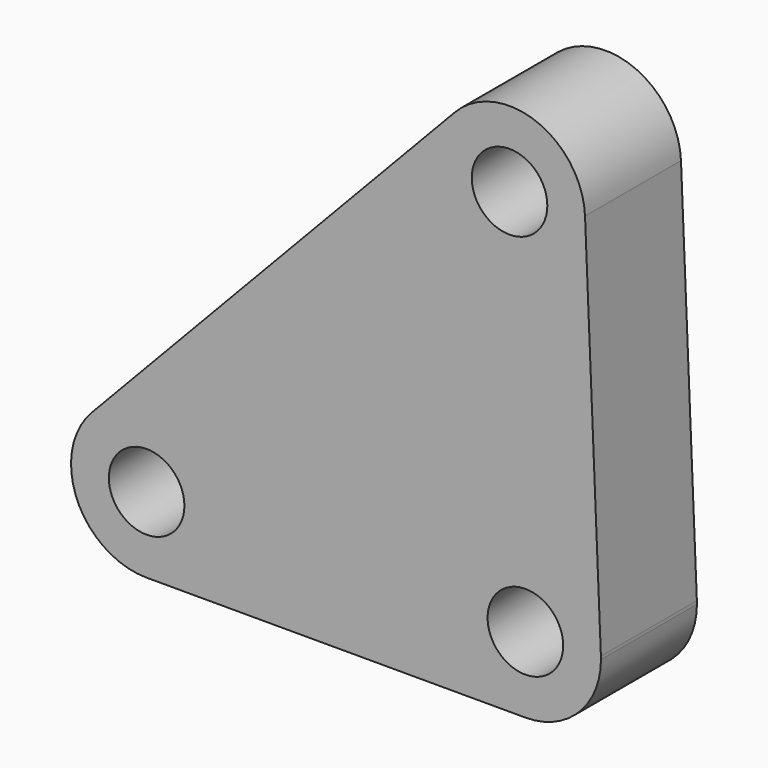
from build123d import *

# Parameters (mm, degrees)
F1_DEPTH = 12.7
F2_R     = 4.0005
F2_R_2   = 4
F3_DEPTH = 12.7


with BuildPart() as f1:
    # F0 (on Front) → F1 (new body)
    with BuildSketch(Plane.XZ):
        with BuildLine():
            Line((-13.8799677983, 7.9941251807), (-13.5483602062, 0))
            Line((-13.5483602062, 0), (-21.5493602062, 0))
            ThreePointArc((-21.5493602062, 0), (-19.2059215625, -5.6575613563), (-13.5483602062, -8.001))
            ThreePointArc((-13.5483602062, -8.001), (-7.8907988499, -5.6575613563), (-5.5473602062, 0))
            ThreePointArc((-5.5473602062, 0), (-5.5490811437, 0.1659381806), (-5.5542432158, 0.3318049778))
            ThreePointArc((-5.5542432158, 0.3318049778), (-8.13021474, 5.8872489932), (-13.8799677983, 7.9941251807))
        make_face()
        with BuildLine():
            Line((-14.8953476758, 32.4720745373), (-13.8799677983, 7.9941251807))
            ThreePointArc((-13.8799677983, 7.9941251807), (-8.13021474, 5.8872489932), (-5.5542432158, 0.3318049778))
            Line((-5.5542432158, 0.3318049778), (-7.2337959714, 40.7969640847))
            ThreePointArc((-7.2337959714, 40.7969640847), (-7.2286345445, 40.6311180182), (-7.2269138221, 40.4652005773))
            ThreePointArc((-7.2269138221, 40.4652005773), (-9.4540233342, 34.9268131392), (-14.8953476758, 32.4720745373))
        make_face()
        with BuildLine():
            Line((-15.2269138221, 40.4652005773), (-14.8953476758, 32.4720745373))
            ThreePointArc((-14.8953476758, 32.4720745373), (-9.4540233342, 34.9268131392), (-7.2269138221, 40.4652005773))
            ThreePointArc((-7.2269138221, 40.4652005773), (-7.2286345445, 40.6311180182), (-7.2337959714, 40.7969640847))
            ThreePointArc((-7.2337959714, 40.7969640847), (-12.4160884571, 47.9551445535), (-21.0282775518, 45.9737556397))
            ThreePointArc((-21.0282775518, 45.9737556397), (-23.2242322391, 40.2580819225), (-20.7353649166, 34.6637381289))
            Line((-20.7353649166, 34.6637381289), (-15.2269138221, 40.4652005773))
        make_face()
        with BuildLine():
            Line((-48.1392205553, 5.8021876312), (-20.7353649166, 34.6637381289))
            ThreePointArc((-20.7353649166, 34.6637381289), (-23.2242322391, 40.2580819225), (-21.0282775518, 45.9737556397))
            Line((-21.0282775518, 45.9737556397), (-59.4504491063, 5.5092436318))
            ThreePointArc((-59.4504491063, 5.5092436318), (-53.8555047508, 7.9983180818), (-48.1392205553, 5.8021876312))
        make_face()
        with BuildLine():
            ThreePointArc((-53.6483602062, -8.001), (-47.9907988499, -5.6575613563), (-45.6473602062, 0))
            Line((-45.6473602062, 0), (-53.6483602062, 0))
            Line((-53.6483602062, 0), (-48.1392205553, 5.8021876312))
            ThreePointArc((-48.1392205553, 5.8021876312), (-53.8555047508, 7.9983180818), (-59.4504491063, 5.5092436318))
            ThreePointArc((-59.4504491063, 5.5092436318), (-61.0000763085, -3.1572569346), (-53.6483602062, -8.001))
        make_face()
        with BuildLine():
            ThreePointArc((-13.5483602062, -8.001), (-19.2059215625, -5.6575613563), (-21.5493602062, 0))
            Line((-21.5493602062, 0), (-45.6473602062, 0))
            ThreePointArc((-45.6473602062, 0), (-47.9907988499, -5.6575613563), (-53.6483602062, -8.001))
            Line((-53.6483602062, -8.001), (-13.5483602062, -8.001))
        make_face()
        with BuildLine():
            ThreePointArc((-21.5493602062, 0), (-19.3219723054, 5.5390797365), (-13.8799677983, 7.9941251807))
            Line((-13.8799677983, 7.9941251807), (-14.8953476758, 32.4720745373))
            ThreePointArc((-14.8953476758, 32.4720745373), (-18.0377645415, 32.975266116), (-20.7353649166, 34.6637381289))
            Line((-20.7353649166, 34.6637381289), (-48.1392205553, 5.8021876312))
            ThreePointArc((-48.1392205553, 5.8021876312), (-46.296672395, 3.15732281), (-45.6473602062, 0))
            Line((-45.6473602062, 0), (-21.5493602062, 0))
        make_face()
        with BuildLine():
            ThreePointArc((-20.7353649166, 34.6637381289), (-18.0377645415, 32.975266116), (-14.8953476758, 32.4720745373))
            Line((-14.8953476758, 32.4720745373), (-15.2269138221, 40.4652005773))
            Line((-15.2269138221, 40.4652005773), (-20.7353649166, 34.6637381289))
        make_face()
        with BuildLine():
            Line((-21.5493602062, 0), (-13.5483602062, 0))
            Line((-13.5483602062, 0), (-13.8799677983, 7.9941251807))
            ThreePointArc((-13.8799677983, 7.9941251807), (-19.3219723054, 5.5390797365), (-21.5493602062, 0))
        make_face()
        with BuildLine():
            Line((-53.6483602062, 0), (-45.6473602062, 0))
            ThreePointArc((-45.6473602062, 0), (-46.296672395, 3.15732281), (-48.1392205553, 5.8021876312))
            Line((-48.1392205553, 5.8021876312), (-53.6483602062, 0))
        make_face()
    extrude(amount=F1_DEPTH)

    # F2 (on face) → F3 (cut, through all)
    with BuildSketch(Plane.XZ.offset(12.7)):
        with Locations((-15.2269138221, 40.4652005773)):
            Circle(F2_R)
        with Locations((-13.5483602062, 0)):
            Circle(F2_R)
        with Locations((-53.6483602062, 0)):
            Circle(F2_R_2)
    extrude(amount=-F3_DEPTH, mode=Mode.SUBTRACT)


solid = f1.part
